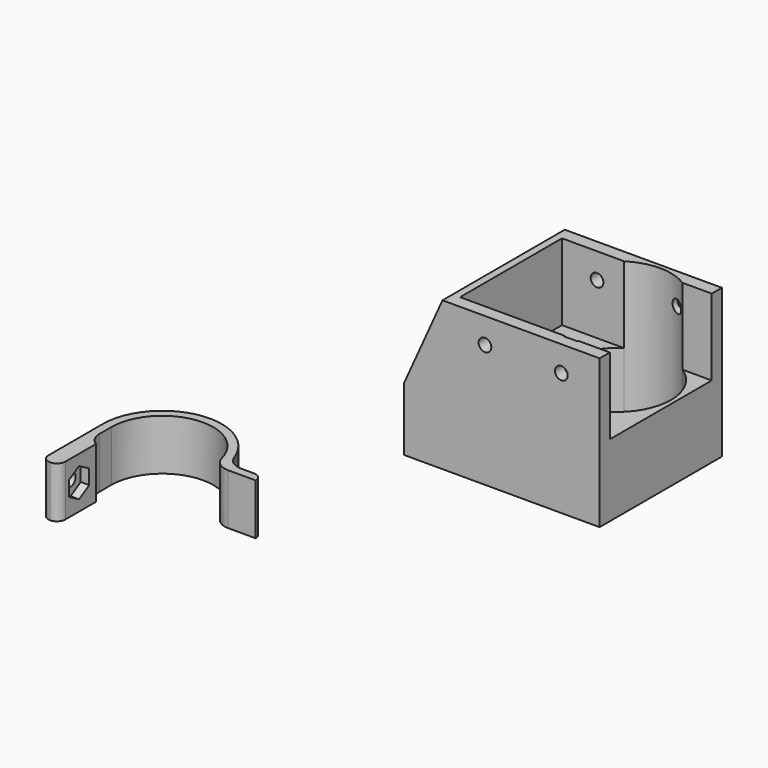
from build123d import *

# Parameters (mm, degrees)
F0_W         = 46
F0_H         = 36
F1_DEPTH     = 35
F2_R         = 1.5
F3_DEPTH     = 50
F2_R_2       = 3
F4_DEPTH     = 30
F6_DEPTH     = 18
F8_DEPTH     = 25
F9_R         = 1.5
F10_DEPTH    = 50
F11_T1_DEPTH = 139.6606830198
F13_DEPTH    = 6
F14_W        = 11
F14_H        = 12
F15_DEPTH    = 2
F14_R        = 1.5
F16_DEPTH    = 25
F17_T1_DEPTH = 12
F17_T3_DEPTH = 12
F17_T5_DEPTH = 29.4596669241
F18_R        = 1.99999


# Not quite as in the source:
# - a fillet or chamfer that OpenCascade refuses, or shapes differently, is made with other operations: its cross-section is extruded or revolved along the edge and cut away or added
# - a fillet or chamfer is up to 0.001 mm smaller than in the source, because OpenCascade refuses the exact size
# - a feature names something its author has since deleted; it is built from what else it names


with BuildPart() as f1:
    # F0 (on Top) → F1 (new body)
    with BuildSketch(Plane.XY):
        Rectangle(F0_W, F0_H)
    extrude(amount=F1_DEPTH)

    # F2 (on face) → F3 (cut)
    with BuildSketch(Plane.XY.offset(35)):
        with Locations((-18, 13)):
            Circle(F2_R)
        with Locations((-18, -13)):
            Circle(F2_R)
        with Locations((14, -12.5)):
            Circle(F2_R)
    extrude(amount=-F3_DEPTH, mode=Mode.SUBTRACT)

    # F2 (on face) → F4 (cut)
    with BuildSketch(Plane.XY.offset(35)):
        with Locations((-18, 13)):
            Circle(F2_R_2)
        with Locations((-18, 13)):
            Circle(F2_R, mode=Mode.SUBTRACT)
        with Locations((-18, -13)):
            Circle(F2_R_2)
        with Locations((-18, -13)):
            Circle(F2_R, mode=Mode.SUBTRACT)
        Polygon((10.8247584463, -12.5342696548), (12.4420576148, -15.266974676), (15.6172991685, -15.2327050212), (17.1752415537, -12.4657303452), (15.5579423852, -9.733025324), (12.3827008315, -9.7672949788), align=None)
        with Locations((14, -12.5)):
            Circle(F2_R, mode=Mode.SUBTRACT)
    extrude(amount=-F4_DEPTH, mode=Mode.SUBTRACT)

    # F5 (on face) → F6 (cut)
    with BuildSketch(Plane.XY.offset(35)):
        Polygon((15.7483235031, -15), (23, -15), (23, 15), (-12.25, 15), (-12.25, -15), (12.2840537621, -15), (10.8247584463, -12.5342696548), (12.3827008315, -9.7672949788), (15.5579423852, -9.733025324), (17.1752415537, -12.4657303452), align=None)
    extrude(amount=-F6_DEPTH, mode=Mode.SUBTRACT)

    # F7 (on face) → F8 (cut, symmetric)
    with BuildSketch(Plane.XY.offset(17)):
        with BuildLine():
            Line((2.3943453996, 15), (16.1056546004, 15))
            ThreePointArc((16.1056546004, 15), (9.25, 17), (2.3943453996, 15))
        make_face()
        with BuildLine():
            ThreePointArc((2.3943453996, 15), (3.120036548, -6.9297159211), (22, 4.25))
            ThreePointArc((22, 4.25), (20.4297159211, 10.379963452), (16.1056546004, 15))
            Line((16.1056546004, 15), (2.3943453996, 15))
        make_face()
    extrude(amount=F8_DEPTH, both=True, mode=Mode.SUBTRACT)

    # F9 (on face) → F10 (cut, symmetric)
    with BuildSketch(Plane.XZ.offset(-15)):
        with Locations((14, 29)):
            Circle(F9_R)
        with Locations((-4, 29)):
            Circle(F9_R)
    extrude(amount=F10_DEPTH, both=True, mode=Mode.SUBTRACT)

    # F11: chamfer of 9 x 20 on 1 edges, made by hand

    # F11_s2 → F11_t1 (cut)
    with BuildSketch(Plane.XZ.offset(-69.8303415099)):
        Polygon((-14, 35), (-23, 15), (-23, 35), align=None)
    extrude(amount=F11_T1_DEPTH, mode=Mode.SUBTRACT)


with BuildPart() as f13:
    # F12 (on Top) → F13 (new body, symmetric)
    with BuildSketch(Plane.XY):
        with BuildLine():
            ThreePointArc((-64.8061240633, -51.9561834335), (-52.8061240633, -39.9561834335), (-40.8061240633, -51.9561834335))
            Line((-40.8061240633, -51.9561834335), (-40.8061240633, -49.9561834335))
            Line((-40.8061240633, -49.9561834335), (-38.9497176027, -49.9561834335))
            ThreePointArc((-38.9497176027, -49.9561834335), (-53.8086981384, -37.9921279616), (-66.8061240633, -51.9561834335))
            Line((-66.8061240633, -51.9561834335), (-64.8061240633, -51.9561834335))
        make_face()
        with BuildLine():
            ThreePointArc((-38.9497176027, -49.9561834335), (-38.8420685913, -50.9536093584), (-38.8061240633, -51.9561834335))
            Line((-38.8061240633, -51.9561834335), (-30.8061240633, -51.9561834335))
            Line((-30.8061240633, -51.9561834335), (-30.8061240633, -49.9561834335))
            Line((-30.8061240633, -49.9561834335), (-38.9497176027, -49.9561834335))
        make_face()
        with BuildLine():
            Line((-40.8061240633, -49.9561834335), (-40.8061240633, -51.9561834335))
            Line((-40.8061240633, -51.9561834335), (-38.8061240633, -51.9561834335))
            ThreePointArc((-38.8061240633, -51.9561834335), (-38.8420685913, -50.9536093584), (-38.9497176027, -49.9561834335))
            Line((-38.9497176027, -49.9561834335), (-40.8061240633, -49.9561834335))
        make_face()
        with BuildLine():
            Line((-64.8061240633, -59.1672859845), (-64.8061240633, -51.9561834335))
            Line((-64.8061240633, -51.9561834335), (-66.8061240633, -51.9561834335))
            ThreePointArc((-66.8061240633, -51.9561834335), (-66.2968616265, -55.6978408203), (-64.8061240633, -59.1672859845))
        make_face()
        with BuildLine():
            ThreePointArc((-64.8061240633, -59.1672859845), (-66.2968616265, -55.6978408203), (-66.8061240633, -51.9561834335))
            Line((-66.8061240633, -51.9561834335), (-66.8061240633, -69.9561834335))
            Line((-66.8061240633, -69.9561834335), (-64.8061240633, -69.9561834335))
            Line((-64.8061240633, -69.9561834335), (-64.8061240633, -59.1672859845))
        make_face()
    extrude(amount=F13_DEPTH, both=True)

    # F14 (on face) → F15 (join)
    with BuildSketch(Plane.YZ.offset(-64.8061240633)):
        with Locations((-64.4561834335, 0)):
            Rectangle(F14_W, F14_H)
        Polygon((-60.9620828312, 1.742268864), (-60.9502840359, -1.7218327511), (-63.9443846382, -3.4641016151), (-66.9502840359, -1.742268864), (-66.9620828312, 1.7218327511), (-63.9679822288, 3.4641016151), align=None, mode=Mode.SUBTRACT)
    extrude(amount=F15_DEPTH)

    # F14 (on face) → F16 (cut)
    with BuildSketch(Plane.YZ.offset(-64.8061240633)):
        with Locations((-63.9561834335, 0)):
            Circle(F14_R)
    extrude(amount=-F16_DEPTH, mode=Mode.SUBTRACT)

    # F17: fillet of radius 4 on 3 edges, made by hand

    # F17_s2 → F17_t1 (join)
    with BuildSketch(Plane.XY.offset(-6)):
        with BuildLine():
            ThreePointArc((-64.8061240633, -55.4920818184), (-64.2702256784, -57.4920818184), (-62.8061240633, -58.9561834335))
            Line((-62.8061240633, -58.9561834335), (-64.8061240633, -58.9561834335))
            Line((-64.8061240633, -58.9561834335), (-64.8061240633, -55.4920818184))
        make_face()
    extrude(amount=F17_T1_DEPTH)

    # F17_s4 → F17_t3 (join)
    with BuildSketch(Plane.XY.offset(-6)):
        with BuildLine():
            ThreePointArc((-35.8355613148, -49.9561834335), (-38.1449623915, -49.2221697572), (-39.6067974811, -47.2895167669))
            ThreePointArc((-39.6067974811, -47.2895167669), (-39.2127083631, -48.6066984578), (-38.9497176027, -49.9561834335))
            Line((-38.9497176027, -49.9561834335), (-35.8355613148, -49.9561834335))
        make_face()
    extrude(amount=F17_T3_DEPTH)

    # F17_s6 → F17_t5 (cut)
    with BuildSketch(Plane.XY.offset(-14.7298334621)):
        with BuildLine():
            ThreePointArc((-41.1871740246, -48.9561834335), (-39.7636804212, -51.1184610937), (-37.3141906784, -51.9561834335))
            Line((-37.3141906784, -51.9561834335), (-40.8061240633, -51.9561834335))
            ThreePointArc((-40.8061240633, -51.9561834335), (-40.9017677081, -50.4441319237), (-41.1871740246, -48.9561834335))
        make_face()
    extrude(amount=F17_T5_DEPTH, mode=Mode.SUBTRACT)

    # F18 (radius 2 in the source; OpenCascade refuses exactly that, so slightly less here)
    f18_edges = [f13.edges().sort_by_distance(p)[0] for p in [
        (-66.806124, -69.956183, 0),
        (-62.806124, -69.956183, 0),
        (-30.806124, -49.956183, 0),
    ]]
    fillet(f18_edges, radius=F18_R)


solid = Compound([f1.part, f13.part])
